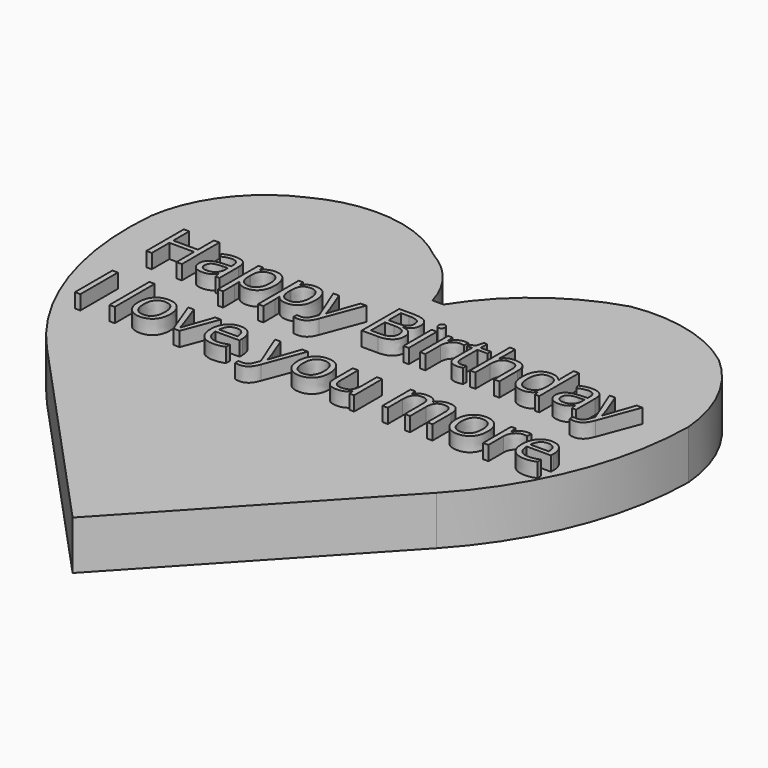
from build123d import *

# Parameters (mm, degrees)
F1_DEPTH     = 12.954
F2_TEXT_SIZE = 17.4069473594
F3_DEPTH     = 3.81


# Not quite as in the source:
# - Text() gives the source's letters only with a copy of the font that has no kerning and outlines rounded to 1/6400 em; it was checked with that copy


with BuildPart() as f1:
    # F0 (on Top) → F1 (new body)
    with BuildSketch(Plane.XY):
        with BuildLine():
            Line((-48.9956966412, -22.2974440235), (2.6404856421, -78.3344378687))
            Line((2.6404856421, -78.3344378687), (54.5590973669, -22.5590153551))
            ThreePointArc((54.5590973669, -22.5590153551), (70.9106831461, 3.2316430076), (76.8565413904, 33.1845925454))
            ThreePointArc((76.8565413904, 33.1845925454), (72.6310206768, 48.1759994182), (63.0673307689, 60.469621369))
            ThreePointArc((63.0673307689, 60.469621369), (49.1607224986, 67.188008855), (33.7285916997, 67.8043066759))
            ThreePointArc((33.7285916997, 67.8043066759), (16.2026802829, 58.8418542788), (2.9338740148, 44.3014999441))
            Line((2.9338740148, 44.3014999441), (0, 44.3014999441))
            ThreePointArc((0, 44.3014999441), (-4.7137449351, 53.6159378813), (-12.615659289, 60.4378067559))
            ThreePointArc((-12.615659289, 60.4378067559), (-30.2285086, 67.8501321318), (-48.9956966412, 64.2518434608))
            ThreePointArc((-48.9956966412, 64.2518434608), (-62.571777714, 53.521847615), (-69.2394282608, 37.5535908431))
            ThreePointArc((-69.2394282608, 37.5535908431), (-65.4708296565, 5.4791742888), (-48.9956966412, -22.2974440235))
        make_face()
    extrude(amount=F1_DEPTH)

    # F2 (on face) → F3 (join)
    with BuildSketch(Plane.XY.offset(12.954)):
        with Locations((-57.2937152997, 18.8890215496)):
            Text('Happy Birthday', F2_TEXT_SIZE, font='Open Sans', text_align=(TextAlign.LEFT, TextAlign.BOTTOM))
        with Locations((-57.2937152997, -4.7844268592)):
            Text('I love you more', F2_TEXT_SIZE, font='Open Sans', text_align=(TextAlign.LEFT, TextAlign.BOTTOM))
    extrude(amount=F3_DEPTH)


solid = f1.part
